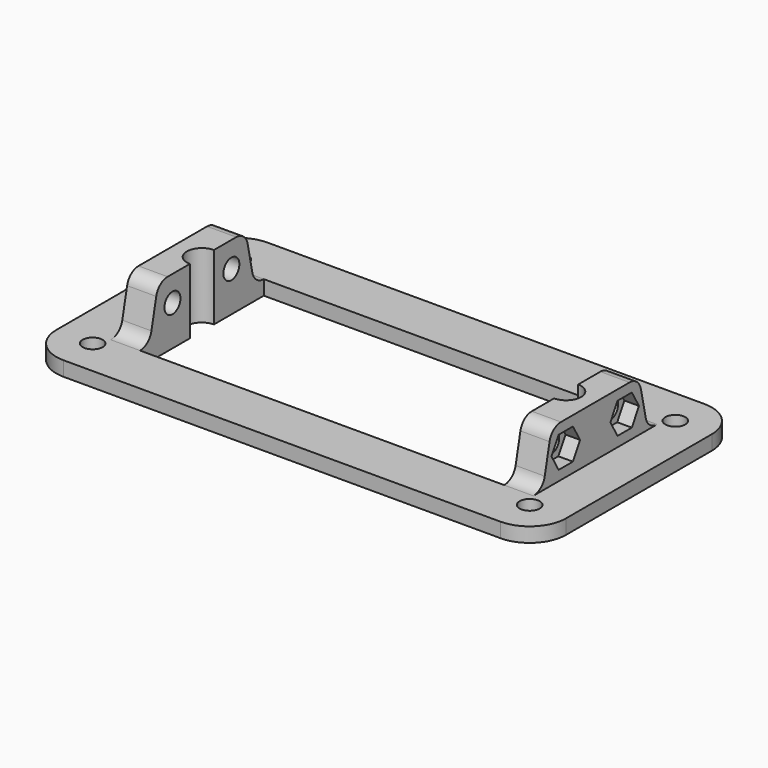
from build123d import *

# Parameters (mm, degrees)
F0_R     = 2.75
F0_W     = 100
F0_H     = 42.47
F1_DEPTH = 4
F2_R     = 2.75
F3_DEPTH = 8
F4_R     = 2.75
F5_DEPTH = 4
F7_R     = 4.125
F8_DEPTH = 18.001


with BuildPart() as f1:
    # F0 (on Top) → F1 (new body)
    with BuildSketch(Plane.XY):
        with BuildLine():
            ThreePointArc((70, 25), (67.0710678119, 32.0710678119), (60, 35))
            Line((60, 35), (-60, 35))
            ThreePointArc((-60, 35), (-67.0710678119, 32.0710678119), (-70, 25))
            Line((-70, 25), (-70, -25))
            ThreePointArc((-70, -25), (-67.0710678119, -32.0710678119), (-60, -35))
            Line((-60, -35), (60, -35))
            ThreePointArc((60, -35), (67.0710678119, -32.0710678119), (70, -25))
            Line((70, -25), (70, 25))
        make_face()
        with Locations((-60, -25)):
            Circle(F0_R, mode=Mode.SUBTRACT)
        with Locations((60, -25)):
            Circle(F0_R, mode=Mode.SUBTRACT)
        with Locations((-60, 25)):
            Circle(F0_R, mode=Mode.SUBTRACT)
        Rectangle(F0_W, F0_H, mode=Mode.SUBTRACT)
        with Locations((60, 25)):
            Circle(F0_R, mode=Mode.SUBTRACT)
    extrude(amount=F1_DEPTH)

    # F2 (on face) → F3 (join)
    with BuildSketch(Plane.YZ.offset(-50)):
        with BuildLine():
            ThreePointArc((-17.3240695981, 7.1605815157), (-18.7208076781, 4.8889170746), (-21.235, 4))
            Line((-21.235, 4), (21.235, 4))
            ThreePointArc((21.235, 4), (18.7208076781, 4.8889170746), (17.3240695981, 7.1605815157))
            Line((17.3240695981, 7.1605815157), (15.6759304019, 14.8394184843))
            ThreePointArc((15.6759304019, 14.8394184843), (14.2791923219, 17.1110829254), (11.765, 18))
            Line((11.765, 18), (-11.765, 18))
            ThreePointArc((-11.765, 18), (-14.2791923219, 17.1110829254), (-15.6759304019, 14.8394184843))
            Line((-15.6759304019, 14.8394184843), (-17.3240695981, 7.1605815157))
        make_face()
        with Locations((-10.11, 11)):
            Circle(F2_R, mode=Mode.SUBTRACT)
        with Locations((10.11, 11)):
            Circle(F2_R, mode=Mode.SUBTRACT)
    extrude(amount=-F3_DEPTH)

    # F4 (on face) → F5 (cut)
    with BuildSketch(Plane(origin=(-58, 0, 0), x_dir=(0, -1, 0), z_dir=(-1, 0, 0))):
        Polygon((-5.2025227119, 11), (-7.6562613559, 15.25), (-12.5637386441, 15.25), (-15.0174772881, 11), (-12.5637386441, 6.75), (-7.6562613559, 6.75), align=None)
        with Locations((-10.11, 11)):
            Circle(F4_R, mode=Mode.SUBTRACT)
        Polygon((7.6562613559, 6.75), (12.5637386441, 6.75), (15.0174772881, 11), (12.5637386441, 15.25), (7.6562613559, 15.25), (5.2025227119, 11), align=None)
        with Locations((10.11, 11)):
            Circle(F4_R, mode=Mode.SUBTRACT)
    extrude(amount=-F5_DEPTH, mode=Mode.SUBTRACT)

    # F6: F1 across plane


with BuildPart() as f1_1:
    add(f1.part)
    add(f1.part.mirror(Plane.YZ))

    # F7 (on face) → F8 (cut, through all)
    with BuildSketch(Plane(origin=(0, 0, 0), x_dir=(1, 0, 0), z_dir=(0, 0, -1))):
        with Locations((-50, 0)):
            Circle(F7_R)
        with Locations((50, 0)):
            Circle(F7_R)
    extrude(amount=-F8_DEPTH, mode=Mode.SUBTRACT)


solid = f1_1.part
